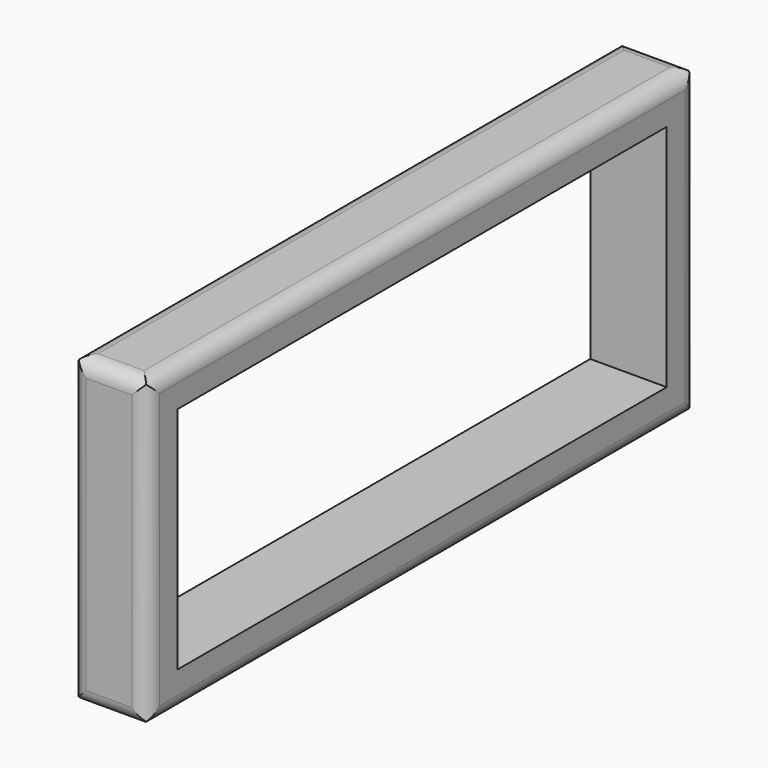
from build123d import *

# Parameters (mm, degrees)
F0_W        = 228.6
F0_H        = 101.6
F0_W_2      = 203.2
F0_H_2      = 76.2
F1_DEPTH    = 25.4
F2_R        = 5.08
F3_T1_DEPTH = 243.84
F4_T1_DEPTH = 243.84


# Not quite as in the source:
# - a fillet or chamfer that OpenCascade refuses, or shapes differently, is made with other operations: its cross-section is extruded or revolved along the edge and cut away or added


with BuildPart() as f1:
    # F0 (on Right) → F1 (new body)
    with BuildSketch(Plane.YZ):
        with Locations((0.4783831537, -17.3432382704)):
            Rectangle(F0_W, F0_H)
        with Locations((0.4783831537, -17.3432382704)):
            Rectangle(F0_W_2, F0_H_2, mode=Mode.SUBTRACT)
    extrude(amount=F1_DEPTH)

    # F2
    f2_edges = [f1.edges().sort_by_distance(p)[0] for p in [
        (12.7, -113.821617, 33.456762),
        (12.7, -113.821617, -68.143238),
        (0, -113.821617, -17.343238),
        (25.4, -113.821617, -17.343238),
        (12.7, 114.778383, -68.143238),
        (12.7, 114.778383, 33.456762),
        (0, 114.778383, -17.343238),
        (25.4, 114.778383, -17.343238),
    ]]
    fillet(f2_edges, radius=F2_R)

    # F3: fillet of radius 5.08 on 4 edges, made by hand

    # F3_s2 → F3_t1 (cut)
    with BuildSketch(Plane.XZ.offset(-122.3983831537)):
        with BuildLine():
            ThreePointArc((0, -63.0632382704), (1.4878975516, -66.6553407189), (5.08, -68.1432382704))
            Line((5.08, -68.1432382704), (0, -68.1432382704))
            Line((0, -68.1432382704), (0, -63.0632382704))
        make_face()
        with BuildLine():
            ThreePointArc((25.4, -63.0632382704), (23.9121024484, -66.6553407189), (20.32, -68.1432382704))
            Line((20.32, -68.1432382704), (25.4, -68.1432382704))
            Line((25.4, -68.1432382704), (25.4, -63.0632382704))
        make_face()
    extrude(amount=F3_T1_DEPTH, mode=Mode.SUBTRACT)

    # F4: fillet of radius 5.08 on 4 edges, made by hand

    # F4_s2 → F4_t1 (cut)
    with BuildSketch(Plane.XZ.offset(-122.3983831537)):
        with BuildLine():
            ThreePointArc((5.08, 33.4567617296), (1.4878975516, 31.968864178), (0, 28.3767617296))
            Line((0, 28.3767617296), (0, 33.4567617296))
            Line((0, 33.4567617296), (5.08, 33.4567617296))
        make_face()
        with BuildLine():
            ThreePointArc((20.32, 33.4567617296), (23.9121024484, 31.968864178), (25.4, 28.3767617296))
            Line((25.4, 28.3767617296), (25.4, 33.4567617296))
            Line((25.4, 33.4567617296), (20.32, 33.4567617296))
        make_face()
    extrude(amount=F4_T1_DEPTH, mode=Mode.SUBTRACT)


solid = f1.part
